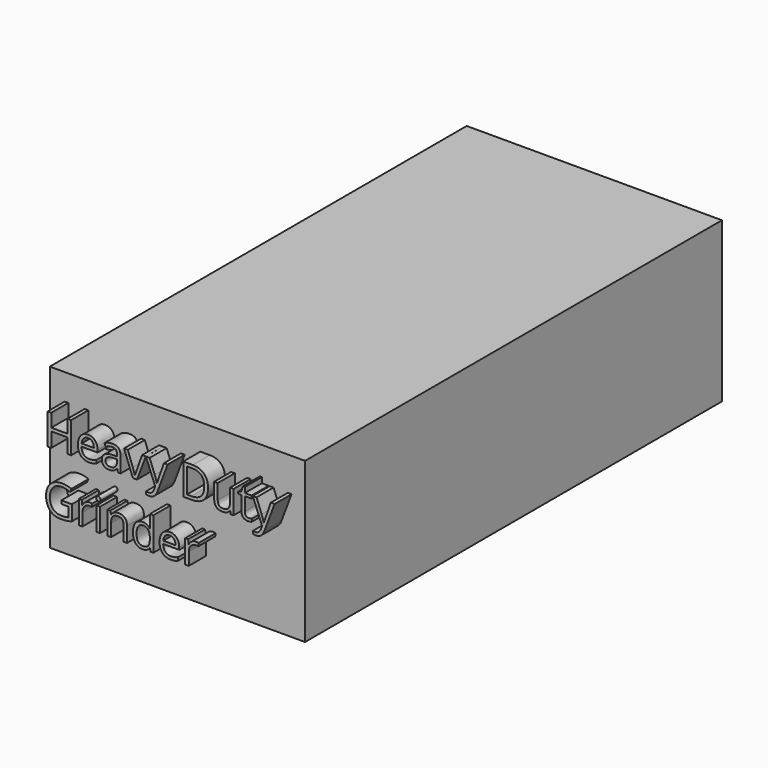
from build123d import *

# Parameters (mm, degrees)
F0_W         = 304.8
F0_H         = 190.5
F1_DEPTH     = 622.3
F2_TEXT_SIZE = 51.9014309349
F3_DEPTH     = 25.4


# Not quite as in the source:
# - Text() gives the source's letters only with a copy of the font that has no kerning and outlines rounded to 1/6400 em; it was checked with that copy


with BuildPart() as f1:
    # F0 (on Front) → F1 (new body)
    with BuildSketch(Plane.XZ):
        Rectangle(F0_W, F0_H)
    extrude(amount=F1_DEPTH)

    # F2 (on face) → F3 (join)
    with BuildSketch(Plane.XZ.offset(622.3)):
        with Locations((-139.7, 27.1962152523)):
            Text('Heavy Duty', F2_TEXT_SIZE, font='Open Sans', text_align=(TextAlign.LEFT, TextAlign.BOTTOM))
        with Locations((-139.7, -43.3897308191)):
            Text('Grinder', F2_TEXT_SIZE, font='Open Sans', text_align=(TextAlign.LEFT, TextAlign.BOTTOM))
    extrude(amount=F3_DEPTH)


solid = f1.part
